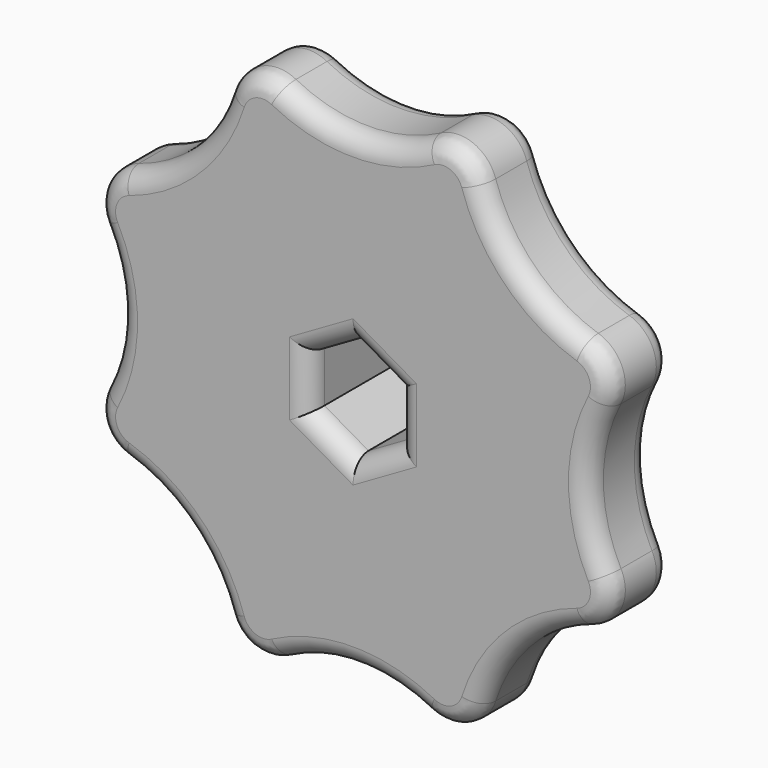
from build123d import *

# Parameters (mm, degrees)
F0_R     = 11.43
F1_DEPTH = 15.24
F3_DEPTH = 8.89
F4_R     = 3.683
F5_DEPTH = 6.351
F6_SIZE2 = 1.27
F6_SIZE  = 5.08
F7_R     = 11.43
F8_DEPTH = 10.16
F9_R     = 5.08
F10_R    = 2.54


with BuildPart() as f1:
    # F0 (on Front) → F1 (new body)
    with BuildSketch(Plane.XZ):
        Circle(F0_R)
    extrude(amount=F1_DEPTH)

    # F2 (on face) → F3 (cut)
    with BuildSketch(Plane.XZ.offset(15.24)):
        Polygon((5.7785, -3.3362185305), (5.7785, 3.3362185305), (0, 6.672437061), (-5.7785, 3.3362185305), (-5.7785, -3.3362185305), (0, -6.672437061), align=None)
    extrude(amount=-F3_DEPTH, mode=Mode.SUBTRACT)

    # F4 (on face) → F5 (cut, through all)
    with BuildSketch(Plane.XZ.offset(6.35)):
        Circle(F4_R)
    extrude(amount=-F5_DEPTH, mode=Mode.SUBTRACT)

    # F6
    f6_edges = [f1.edges().sort_by_distance(p)[0] for p in [
        (-11.43, 0, 0),
    ]]
    f6_side = f1.faces().sort_by_distance((-11.43, -7.62, 0))[0]
    chamfer(f6_edges, length=F6_SIZE, length2=F6_SIZE2, reference=f6_side)

    # F7 (on face) → F8 (join)
    with BuildSketch(Plane.XZ.offset(15.24)):
        with BuildLine():
            ThreePointArc((38.1, -15.7815367264), (30.798190085, 0), (38.1, 15.7815367264))
            ThreePointArc((38.1, 15.7815367264), (21.7776090573, 21.7776090573), (15.7815367264, 38.1))
            ThreePointArc((15.7815367264, 38.1), (0, 30.798190085), (-15.7815367264, 38.1))
            ThreePointArc((-15.7815367264, 38.1), (-21.7776090573, 21.7776090573), (-38.1, 15.7815367264))
            ThreePointArc((-38.1, 15.7815367264), (-30.798190085, 0), (-38.1, -15.7815367264))
            ThreePointArc((-38.1, -15.7815367264), (-21.7776090573, -21.7776090573), (-15.7815367264, -38.1))
            ThreePointArc((-15.7815367264, -38.1), (0, -30.798190085), (15.7815367264, -38.1))
            ThreePointArc((15.7815367264, -38.1), (21.7776090573, -21.7776090573), (38.1, -15.7815367264))
        make_face()
        Circle(F7_R, mode=Mode.SUBTRACT)
        Circle(F7_R)
        Polygon((0, 6.672437061), (5.7785, 3.3362185305), (5.7785, -3.3362185305), (0, -6.672437061), (-5.7785, -3.3362185305), (-5.7785, 3.3362185305), align=None, mode=Mode.SUBTRACT)
    extrude(amount=F8_DEPTH)

    # F9
    f9_edges = [f1.edges().sort_by_distance(p)[0] for p in [
        (-15.781537, -20.32, 38.1),
        (-38.1, -20.32, 15.781537),
        (-38.1, -20.32, -15.781537),
        (-15.781537, -20.32, -38.1),
        (15.781537, -20.32, -38.1),
        (38.1, -20.32, -15.781537),
        (38.1, -20.32, 15.781537),
        (15.781537, -20.32, 38.1),
    ]]
    fillet(f9_edges, radius=F9_R)

    # F10
    f10_edges = [f1.edges().sort_by_distance(p)[0] for p in [
        (0, -25.4, -30.79819),
        (-13.790856, -25.4, -33.294073),
        (13.790856, -25.4, -33.294073),
        (-21.777609, -25.4, -21.777609),
        (21.777609, -25.4, -21.777609),
        (-33.294073, -25.4, -13.790856),
        (33.294073, -25.4, -13.790856),
        (-30.79819, -25.4, 0),
        (30.79819, -25.4, 0),
        (-33.294073, -25.4, 13.790856),
        (33.294073, -25.4, 13.790856),
        (-21.777609, -25.4, 21.777609),
        (21.777609, -25.4, 21.777609),
        (-13.790856, -25.4, 33.294073),
        (13.790856, -25.4, 33.294073),
        (0, -25.4, 30.79819),
        (-5.7785, -25.4, 0),
        (-2.88925, -25.4, 5.004328),
        (2.88925, -25.4, 5.004328),
        (5.7785, -25.4, 0),
        (2.88925, -25.4, -5.004328),
        (-2.88925, -25.4, -5.004328),
        (0, -15.24, -30.79819),
        (-13.790856, -15.24, -33.294073),
        (13.790856, -15.24, -33.294073),
        (-21.777609, -15.24, -21.777609),
        (21.777609, -15.24, -21.777609),
        (-33.294073, -15.24, -13.790856),
        (33.294073, -15.24, -13.790856),
        (-30.79819, -15.24, 0),
        (30.79819, -15.24, 0),
        (-33.294073, -15.24, 13.790856),
        (33.294073, -15.24, 13.790856),
        (-21.777609, -15.24, 21.777609),
        (21.777609, -15.24, 21.777609),
        (-13.790856, -15.24, 33.294073),
        (13.790856, -15.24, 33.294073),
        (0, -15.24, 30.79819),
        (-11.43, -15.24, 0),
    ]]
    fillet(f10_edges, radius=F10_R)


solid = f1.part
